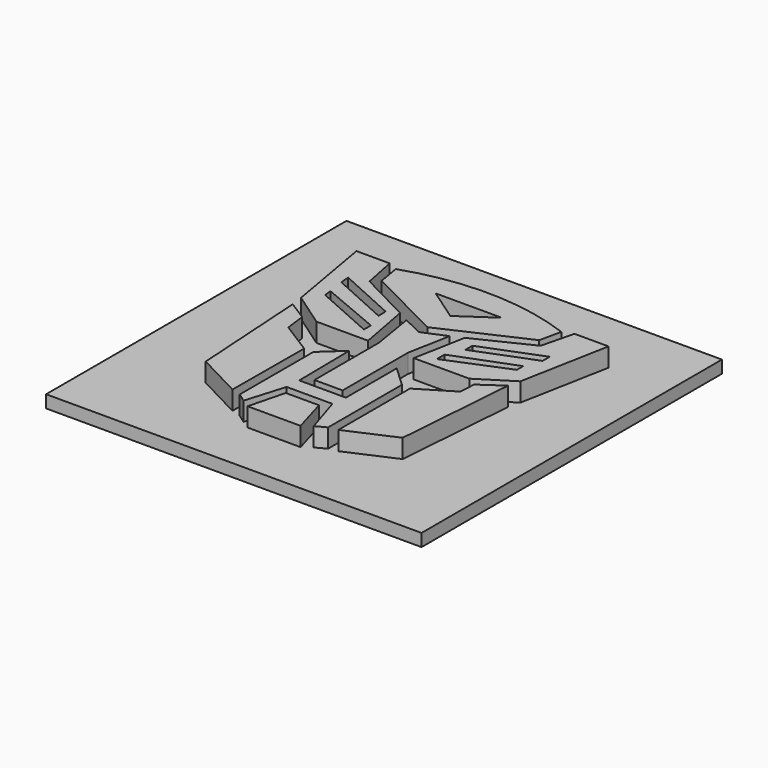
from build123d import *

# Parameters (mm, degrees)
F2_DEPTH = 5
F1_W     = 60
F1_H     = 60
F3_DEPTH = 2


# Not quite as in the source:
# - ends of sketch curves that miss each other by under 0.0002 mm in the source are joined


with BuildPart() as f2:
    # F0 (on Top) → F2 (new body)
    with BuildSketch(Plane.XY):
        with BuildLine():
            Line((12.5301, 15.3483), (13.2754, 18.8292))
            ThreePointArc((13.2754, 18.8292), (-0.0620714554, 21.313337159), (-13.4587020592, 19.1710971727))
            Line((-13.4587020592, 19.1710971727), (-12.8601, 15.6049))
            Line((-12.8601, 15.6049), (-0.5682, 9.3636))
            Line((-0.5682, 9.3636), (12.5301, 15.3483))
        make_face()
        Polygon((5.0768, 17.1559), (-0.2261, 13.5284), (-5.468, 17.1559), align=None, mode=Mode.SUBTRACT)
    extrude(amount=F2_DEPTH)



with BuildPart() as f2b:
    # F0 (on Top) → F2, piece 2 (new body)
    with BuildSketch(Plane.XY):
        Polygon((20.3255, 19.4397), (14.8884, 19.4397), (13.6053, 14.2734), (4.869, 10.0354), (3.3296, 1.7791), (12.2, 1.7791), (17.6374, 5.1989), align=None)
        Polygon((15.3523, 8.6188), (15.3523, 7.3484), (5.7369, 3.3912), (5.7369, 4.9303), align=None, mode=Mode.SUBTRACT)
        Polygon((16.3548, 12.6613), (16.3548, 11.2445), (6.9587, 7.5562), (6.9587, 8.9606), align=None, mode=Mode.SUBTRACT)
    extrude(amount=F2_DEPTH)


with BuildPart() as f2c:
    # F0 (on Top) → F2, piece 3 (new body)
    with BuildSketch(Plane.XY):
        Polygon((-4.0627, 1.9012), (-5.6145, 10.2308), (-13.9352, 14.5301), (-15.0105, 19.9041), (-20.3255, 19.9041), (-17.8452, 5.7363), (-12.3223, 1.9012), align=None)
        Polygon((-16.098, 9.4248), (-6.3597, 5.3332), (-6.3597, 3.9288), (-15.9514, 8.1913), align=None, mode=Mode.SUBTRACT)
        Polygon((-16.6601, 13.6628), (-7.2887, 9.4248), (-7.2152, 7.947), (-16.5379, 12.1483), align=None, mode=Mode.SUBTRACT)
    extrude(amount=F2_DEPTH)


with BuildPart() as f2d:
    # F0 (on Top) → F2, piece 4 (new body)
    with BuildSketch(Plane.XY):
        Polygon((-14.0697, -1.5185), (-14.4852, 1.7669), (-17.5644, 3.7209), (-16.3667, -15.1486), (-9.0357, -18.9712), (-8.9623, -4.7428), align=None)
    extrude(amount=F2_DEPTH)


with BuildPart() as f2e:
    # F0 (on Top) → F2, piece 5 (new body)
    with BuildSketch(Plane.XY):
        Polygon((17.161, 3.318), (13.6663, 0.8999), (13.5321, -1.6531), (8.0952, -4.938), (8.0952, -19.2404), (15.6947, -15.8937), align=None)
    extrude(amount=F2_DEPTH)


with BuildPart() as f2f:
    # F0 (on Top) → F2, piece 6 (new body)
    with BuildSketch(Plane.XY):
        Polygon((-3.794, 9.2295), (-2.6575, 2.3167), (-2.6575, -10.5809), (1.8513, -10.5809), (1.8513, 2.4509), (3.1219, 9.2295), (-0.5682, 7.6783), align=None)
    extrude(amount=F2_DEPTH)


with BuildPart() as f2g:
    # F0 (on Top) → F2, piece 7 (new body)
    with BuildSketch(Plane.XY):
        Polygon((-7.4959, -4.7428), (-7.4959, -19.4476), (-6.0788, -20.4494), (-4.1971, -14.2084), (3.1219, -14.2084), (5.0647, -20.3757), (6.6777, -19.5086), (6.6777, -4.7428), (3.3906, -1.7137), (3.3906, -11.8511), (-4.0627, -11.8511), (-4.1971, -1.7137), align=None)
    extrude(amount=F2_DEPTH)


with BuildPart() as f2h:
    # F0 (on Top) → F2, piece 8 (new body)
    with BuildSketch(Plane.XY):
        Polygon((-3.2564, -15.5518), (-4.7349, -21.3286), (3.7325, -21.3286), (2.047, -15.5518), align=None)
    extrude(amount=F2_DEPTH)


with BuildPart() as f2_1:
    add(f2.part)

    add(f2b.part)  # F3 merges F2b

    add(f2c.part)  # F3 merges F2c

    add(f2d.part)  # F3 merges F2d

    add(f2e.part)  # F3 merges F2e

    add(f2f.part)  # F3 merges F2f

    add(f2g.part)  # F3 merges F2g

    add(f2h.part)  # F3 merges F2h
    # F1 (on Top) → F3 (join)
    with BuildSketch(Plane.XY):
        Rectangle(F1_W, F1_H)
    extrude(amount=F3_DEPTH)


solid = f2_1.part
